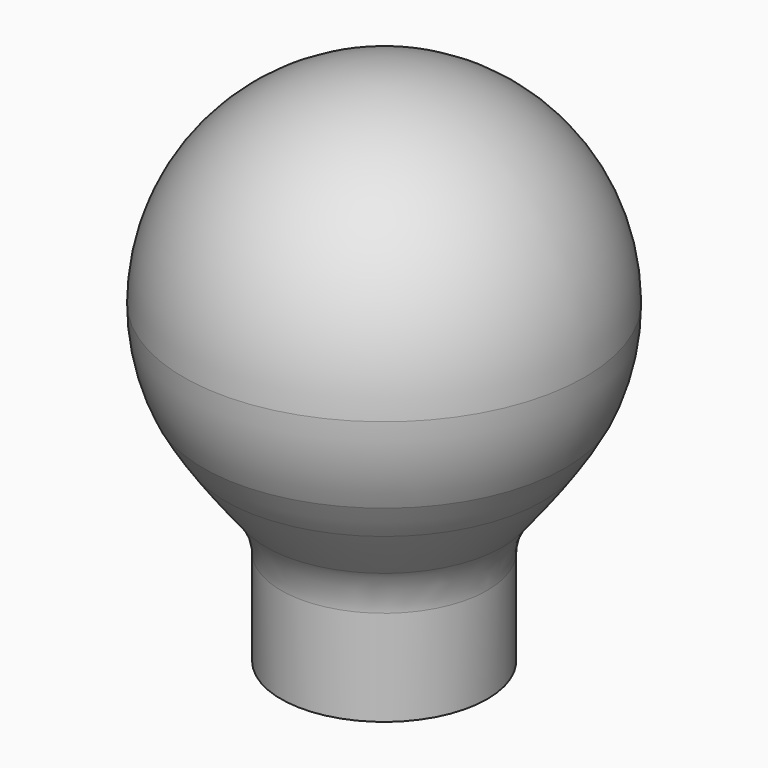
from build123d import *


with BuildPart() as f1:
    # F0 (on Front) → F1 (revolve)
    with BuildSketch(Plane.XZ):
        with BuildLine():
            Line((0, 17.4324345394), (0, 0))
            Line((0, 0), (15, 0))
            Line((15, 0), (15, 13.903540875))
            ThreePointArc((15, 13.903540875), (15.5646049408, 17.2161410738), (17.1946640153, 20.1546791847))
            add(Edge.make_bspline(
                [(17.1946640153, 20.1546791847), (19.2820687523, 22.7610677336), (21.3061725207, 25.3630195661), (23.0850826912, 27.947785967)],
                knots=[0.0438155979, 0.0438155979, 0.0438155979, 0.0438155979, 0.1697178469, 0.1697178469, 0.1697178469, 0.1697178469], degree=3))
            add(Edge.make_bspline(
                [(23.0850826912, 27.947785967), (24.3132478505, 29.7323167944), (25.4245398901, 31.5086560743), (26.3591006498, 33.272608394)],
                knots=[0.1697178469, 0.1697178469, 0.1697178469, 0.1697178469, 0.2566411543, 0.2566411543, 0.2566411543, 0.2566411543], degree=3))
            ThreePointArc((26.3591006498, 33.272608394), (28.4728772846, 39.383993976), (29.1891884869, 45.8108115131))
            add(Edge.make_bspline(
                [(29.1891884869, 45.8108115131), (27.5186066734, 56.1054005015), (13.7593033367, 65.5527002508), (0, 75)],
                knots=[0.4671507953, 0.4671507953, 0.4671507953, 0.4671507953, 1, 1, 1, 1], degree=3))
            Line((0, 75), (0, 17.4324345394))
        make_face()
        with BuildLine():
            ThreePointArc((29.1891884869, 45.8108115131), (20.6398731164, 66.4506846295), (0, 75))
            add(Edge.make_bspline(
                [(29.1891884869, 45.8108115131), (27.5186066734, 56.1054005015), (13.7593033367, 65.5527002508), (0, 75)],
                knots=[0.4671507953, 0.4671507953, 0.4671507953, 0.4671507953, 1, 1, 1, 1], degree=3))
        make_face()
    revolve(axis=Axis((0, 0, 37.5), (0, 0, 1)))


solid = f1.part
